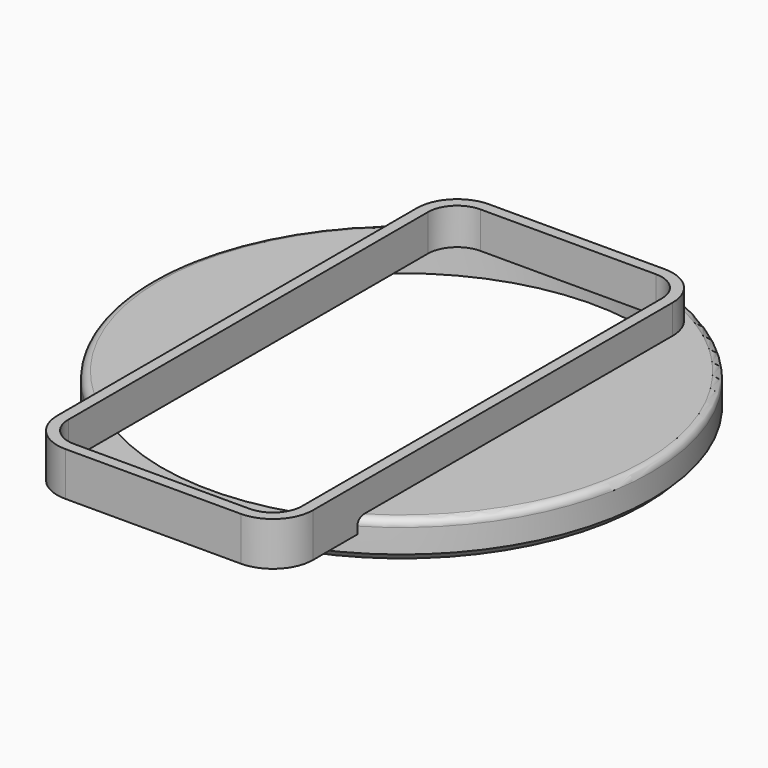
from build123d import *
from build123d import SkipClean  # not in build123d's __all__

# Parameters (mm, degrees)
F0_R     = 68.5
F0_R_2   = 65.5
F1_DEPTH = 2
F2_DEPTH = 8.5
F3_SIZE  = 2
F5_DEPTH = 2
F6_DEPTH = 3
F7_DEPTH = 10
F8_DEPTH = 25
F9_R     = 2


# Not quite as in the source:
# - after a boolean that leaves OpenCascade's solid faulty, fix() repairs it


with BuildPart() as f1:
    # F0 (on Top) → F1 (new body)
    with BuildSketch(Plane.XY):
        Circle(F0_R)
        Circle(F0_R_2, mode=Mode.SUBTRACT)
        Circle(F0_R_2)
    extrude(amount=F1_DEPTH)

    # F0 (on Top) → F2 (join)
    with BuildSketch(Plane.XY):
        Circle(F0_R)
        Circle(F0_R_2, mode=Mode.SUBTRACT)
    extrude(amount=-F2_DEPTH)

    # F3
    f3_edges = [f1.edges().sort_by_distance(p)[0] for p in [
        (-68.5, 0, -8.5),
    ]]
    chamfer(f3_edges, length=F3_SIZE)

    # F4 (on Top) → F5 (join)
    with BuildSketch(Plane.XY):
        with BuildLine():
            Line((35, -74), (35, 49))
            ThreePointArc((35, 49), (31.7781745931, 56.7781745931), (24, 60))
            Line((24, 60), (-24, 60))
            ThreePointArc((-24, 60), (-31.7781745931, 56.7781745931), (-35, 49))
            Line((-35, 49), (-35, -74))
            ThreePointArc((-35, -74), (-31.7781745931, -81.7781745931), (-24, -85))
            Line((-24, -85), (24, -85))
            ThreePointArc((24, -85), (31.7781745931, -81.7781745931), (35, -74))
        make_face()
        with BuildLine():
            ThreePointArc((-32, 49), (-29.6568542495, 54.6568542495), (-24, 57))
            Line((-24, 57), (0, 57))
            Line((0, 57), (24, 57))
            ThreePointArc((24, 57), (29.6568542495, 54.6568542495), (32, 49))
            Line((32, 49), (32, -74))
            ThreePointArc((32, -74), (29.6568542495, -79.6568542495), (24, -82))
            Line((24, -82), (-24, -82))
            ThreePointArc((-24, -82), (-29.6568542495, -79.6568542495), (-32, -74))
            Line((-32, -74), (-32, 49))
        make_face(mode=Mode.SUBTRACT)
        with BuildLine():
            Line((0, 57), (-24, 57))
            ThreePointArc((-24, 57), (-29.6568542495, 54.6568542495), (-32, 49))
            Line((-32, 49), (-32, -74))
            ThreePointArc((-32, -74), (-29.6568542495, -79.6568542495), (-24, -82))
            Line((-24, -82), (24, -82))
            ThreePointArc((24, -82), (29.6568542495, -79.6568542495), (32, -74))
            Line((32, -74), (32, 49))
            ThreePointArc((32, 49), (29.6568542495, 54.6568542495), (24, 57))
            Line((24, 57), (0, 57))
        make_face()
    extrude(amount=-F5_DEPTH)

    # F4 (on Top) → F6 (cut)
    with BuildSketch(Plane.XY):
        with BuildLine():
            Line((0, 57), (-24, 57))
            ThreePointArc((-24, 57), (-29.6568542495, 54.6568542495), (-32, 49))
            Line((-32, 49), (-32, -74))
            ThreePointArc((-32, -74), (-29.6568542495, -79.6568542495), (-24, -82))
            Line((-24, -82), (24, -82))
            ThreePointArc((24, -82), (29.6568542495, -79.6568542495), (32, -74))
            Line((32, -74), (32, 49))
            ThreePointArc((32, 49), (29.6568542495, 54.6568542495), (24, 57))
            Line((24, 57), (0, 57))
        make_face()
    extrude(amount=F6_DEPTH, mode=Mode.SUBTRACT)

    # F4 (on Top) → F7 (join)
    with BuildSketch(Plane.XY):
        with BuildLine():
            Line((35, -74), (35, 49))
            ThreePointArc((35, 49), (31.7781745931, 56.7781745931), (24, 60))
            Line((24, 60), (-24, 60))
            ThreePointArc((-24, 60), (-31.7781745931, 56.7781745931), (-35, 49))
            Line((-35, 49), (-35, -74))
            ThreePointArc((-35, -74), (-31.7781745931, -81.7781745931), (-24, -85))
            Line((-24, -85), (24, -85))
            ThreePointArc((24, -85), (31.7781745931, -81.7781745931), (35, -74))
        make_face()
        with BuildLine():
            ThreePointArc((-32, 49), (-29.6568542495, 54.6568542495), (-24, 57))
            Line((-24, 57), (0, 57))
            Line((0, 57), (24, 57))
            ThreePointArc((24, 57), (29.6568542495, 54.6568542495), (32, 49))
            Line((32, 49), (32, -74))
            ThreePointArc((32, -74), (29.6568542495, -79.6568542495), (24, -82))
            Line((24, -82), (-24, -82))
            ThreePointArc((-24, -82), (-29.6568542495, -79.6568542495), (-32, -74))
            Line((-32, -74), (-32, 49))
        make_face(mode=Mode.SUBTRACT)
    with SkipClean():  # cleaning this boolean's faces spoils the solid; the shape is the same uncleaned
        extrude(amount=F7_DEPTH)

    # F0 (on Top) → F8 (cut)
    with BuildSketch(Plane.XY):
        Circle(F0_R_2)
    extrude(amount=-F8_DEPTH, mode=Mode.SUBTRACT)

    add(f1.part.fix(), mode=Mode.REPLACE)

    # F9
    f9_edges = [f1.edges().sort_by_distance(p)[0] for p in [
        (-33.872924, 59.538853, 2),
    ]]
    fillet(f9_edges, radius=F9_R)


solid = f1.part
